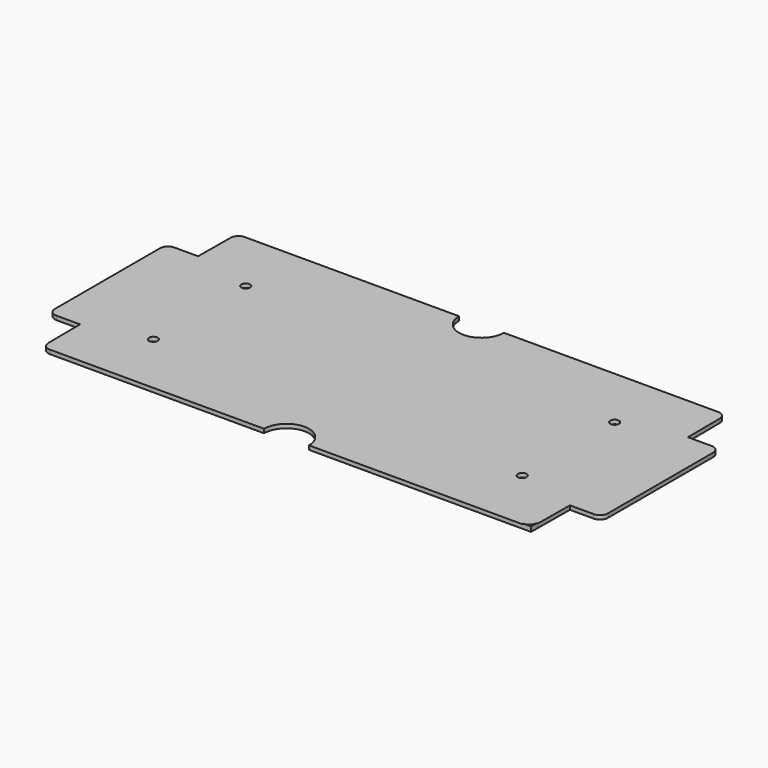
from build123d import *

# Parameters (mm, degrees)
F1_DEPTH = 3
F2_DEPTH = 2.5
F3_D     = 28
F3_DEPTH = 50.5
F3_TIP   = 8.4120486664
F4_D     = 28
F4_DEPTH = 50.5
F4_TIP   = 8.4120486664
F5_D     = 5.5
F5_DEPTH = 14.4
F5_TIP   = 1.6523667023


with BuildPart() as f1:
    # F0 (on Top) → F1 (new body)
    with BuildSketch(Plane.XY):
        with BuildLine():
            ThreePointArc((152.5413805678, -71.0417273613), (151.062304835, -74.5502561039), (147.5415546881, -76))
            Line((147.5415546881, -76), (152.5, -76))
            Line((152.5, -76), (152.5413805678, -71.0417273613))
        make_face()
    extrude(amount=F1_DEPTH)

    # F0 (on Top) → F2 (join)
    with BuildSketch(Plane.XY):
        with BuildLine():
            ThreePointArc((-152.5413805678, -71.0417273613), (-151.062304835, -74.5502561039), (-147.5415546881, -76))
            Line((-147.5415546881, -76), (147.5415546881, -76))
            ThreePointArc((147.5415546881, -76), (151.062304835, -74.5502561039), (152.5413805678, -71.0417273613))
            Line((152.5413805678, -71.0417273613), (152.7503728867, -46))
            Line((152.7503728867, -46), (167.5, -46))
            ThreePointArc((167.5, -46), (171.0355339059, -44.5355339059), (172.5, -41))
            Line((172.5, -41), (172.5, 41))
            ThreePointArc((172.5, 41), (171.0355339059, 44.5355339059), (167.5, 46))
            Line((167.5, 46), (152.7503728867, 46))
            Line((152.7503728867, 46), (152.5413805678, 71.0417273613))
            ThreePointArc((152.5413805678, 71.0417273613), (151.062304835, 74.5502561039), (147.5415546881, 76))
            Line((147.5415546881, 76), (-147.5415546881, 76))
            ThreePointArc((-147.5415546881, 76), (-151.062304835, 74.5502561039), (-152.5413805678, 71.0417273613))
            Line((-152.5413805678, 71.0417273613), (-152.7503728867, 46))
            Line((-152.7503728867, 46), (-167.5, 46))
            ThreePointArc((-167.5, 46), (-171.0355339059, 44.5355339059), (-172.5, 41))
            Line((-172.5, 41), (-172.5, -41))
            ThreePointArc((-172.5, -41), (-171.0355339059, -44.5355339059), (-167.5, -46))
            Line((-167.5, -46), (-152.7503728867, -46))
            Line((-152.7503728867, -46), (-152.5413805678, -71.0417273613))
        make_face()
    extrude(amount=F2_DEPTH)

    # F3
    with Locations(Plane(origin=(0, 0, 0), x_dir=(1, 0, 0), z_dir=(0, 0, -1))):
        with Locations((0, -76)):
            Hole(F3_D / 2, depth=F3_DEPTH)
            with Locations((0, 0, -(F3_DEPTH + F3_TIP / 2))):  # 118° drill point
                Cone(0, F3_D / 2, F3_TIP, mode=Mode.SUBTRACT)

    # F4
    with Locations(Plane(origin=(0, 0, 0), x_dir=(1, 0, 0), z_dir=(0, 0, -1))):
        with Locations((0, 76)):
            Hole(F4_D / 2, depth=F4_DEPTH)
            with Locations((0, 0, -(F4_DEPTH + F4_TIP / 2))):  # 118° drill point
                Cone(0, F4_D / 2, F4_TIP, mode=Mode.SUBTRACT)

    # F5
    with Locations(Plane(origin=(0, 0, 0), x_dir=(1, 0, 0), z_dir=(0, 0, -1))):
        with Locations((-115, 36), (-115, -36), (115, -36), (115, 36)):
            Hole(F5_D / 2, depth=F5_DEPTH)
            with Locations((0, 0, -(F5_DEPTH + F5_TIP / 2))):  # 118° drill point
                Cone(0, F5_D / 2, F5_TIP, mode=Mode.SUBTRACT)


solid = f1.part
